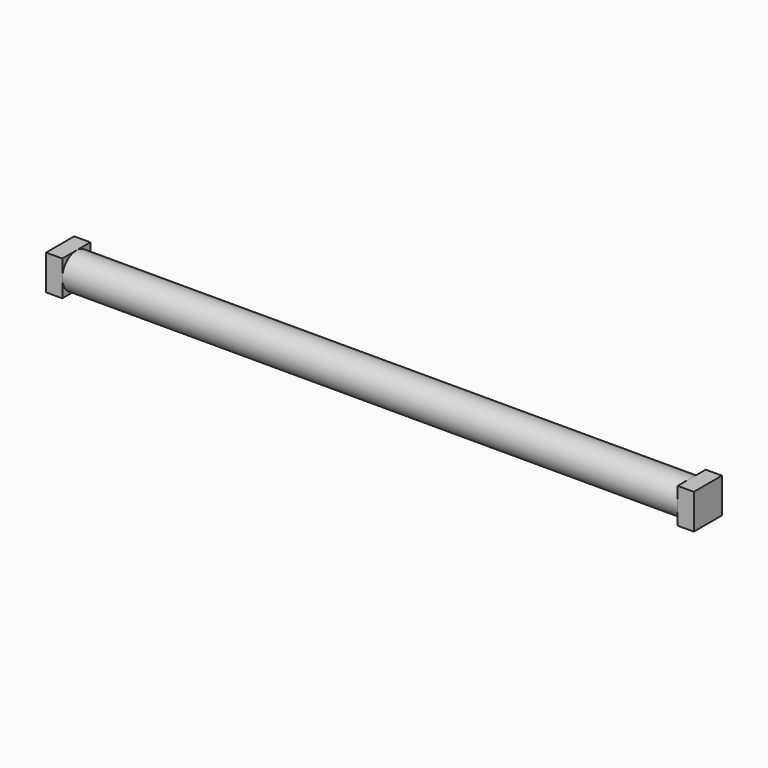
from build123d import *

# Parameters (mm, degrees)
F0_R     = 20.6375
F0_R_2   = 17.4625
F1_DEPTH = 381
F2_W     = 41.275
F2_H     = 41.275
F3_DEPTH = 19.05


# Not quite as in the source:
# - a pattern or mirror of a feature is missing from the dataset's text; its kind, count and spacing are read off the source's solid


with BuildPart() as f1:
    # F0 (on Right) → F1 (new body, symmetric)
    with BuildSketch(Plane.YZ):
        Circle(F0_R)
        Circle(F0_R_2, mode=Mode.SUBTRACT)
    extrude(amount=F1_DEPTH, both=True)

    # F2 (on face) → F3 (join)
    with BuildSketch(Plane(origin=(-381, 0, 0), x_dir=(0, -1, 0), z_dir=(-1, 0, 0))):
        Rectangle(F2_W, F2_H)
    f3 = extrude(amount=-F3_DEPTH)

    # F3_copies: F3 across plane
    add(f3.mirror(Plane(origin=(0, 0, 0), x_dir=(0, 0, 1), z_dir=(1, 0, 0))))


solid = f1.part
